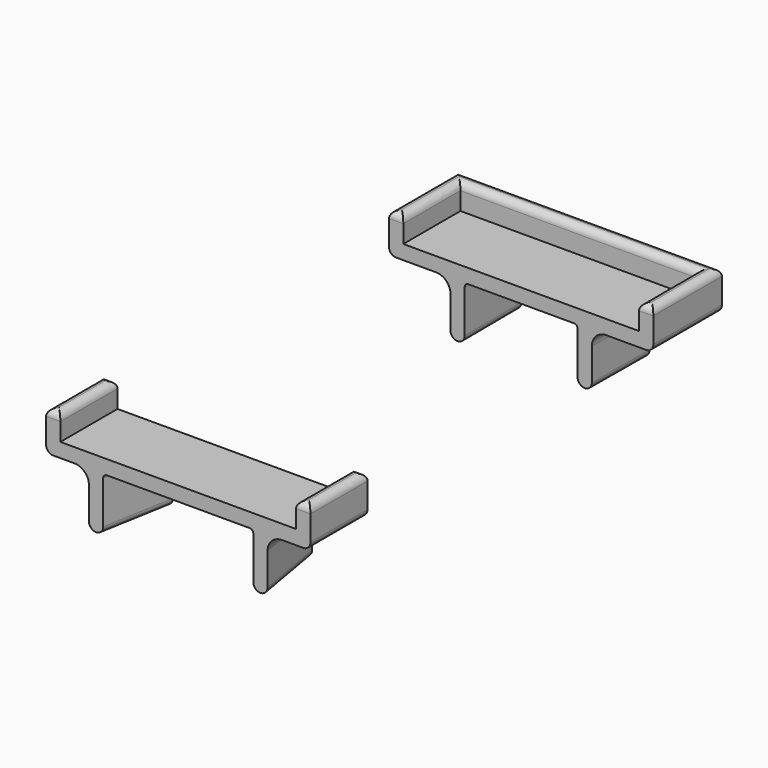
from build123d import *

# Parameters (mm, degrees)
F10_W        = 74
F10_H        = 11
F11_DEPTH    = 4
F12_R        = 1.99999
F12_2_R      = 1.99999
F13_R        = 4
F13_2_R      = 4
F14_R        = 1
F14_2_R      = 1
F15_T1_DEPTH = 30.3039405042
F15_T3_DEPTH = 30.3039405042
F15_T5_DEPTH = 30.3039405042
F15_T7_DEPTH = 30.3039405042
F15_2_F1_R   = 2
F15_2_F2_R   = 1.9999
F15_2_F3_R   = 2
F15_2_F4_R   = 1.9999


# Not quite as in the source:
# - a fillet or chamfer that OpenCascade refuses, or shapes differently, is made with other operations: its cross-section is extruded or revolved along the edge and cut away or added
# - a fillet or chamfer is up to 0.001 mm smaller than in the source, because OpenCascade refuses the exact size


with BuildPart() as f8:
    # F0 (on Front) → F8 section 0
    with BuildSketch(Plane.XZ):
        Polygon((-33, 11), (-37, 11), (-37, 0), (-19.95, 0), (-19.95, -15), (-15.95, -15), (-15.95, 0), (15.95, 0), (15.95, -15), (19.95, -15), (19.95, 0), (37, 0), (37, 11), (33, 11), (33, 4), (-33, 4), align=None)
    # F3 (on plane+point) → F8 section 1
    with BuildSketch(Plane.XZ.offset(20)):
        Polygon((-33, 11), (-37, 11), (-37, 0), (-19.8, 0), (-19.8, -15), (-15.8, -15), (-15.8, 0), (15.8, 0), (15.8, -15), (19.8, -15), (19.8, 0), (37, 0), (37, 11), (33, 11), (33, 4), (-33, 4), align=None)
    loft()

    # F10 (on face) → F11 (join)
    with BuildSketch(Plane(origin=(0, 0, 0), x_dir=(-1, 0, 0), z_dir=(0, 1, 0))):
        with Locations((0, 5.5)):
            Rectangle(F10_W, F10_H)
    extrude(amount=F11_DEPTH)

    # F12 (radius 2 in the source; OpenCascade refuses exactly that, so slightly less here)
    f12_edges = [f8.edges().sort_by_distance(p)[0] for p in [
        (-35, -20, 11),
        (-33, -10, 11),
        (0, 0, 11),
        (33, -10, 11),
        (35, -20, 11),
        (37, -8, 11),
        (0, 4, 11),
        (-37, -8, 11),
        (-37, -8, 0),
        (37, -8, 0),
    ]]
    fillet(f12_edges, radius=F12_R)

    # F13#2
    f13_2_edges = [f8.edges().sort_by_distance(p)[0] for p in [
        (-19.875, -10, 0),
        (19.875, -10, 0),
    ]]
    fillet(f13_2_edges, radius=F13_2_R)

    # F14#2
    f14_2_edges = [f8.edges().sort_by_distance(p)[0] for p in [
        (15.875, -10, 0),
        (-15.875, -10, 0),
    ]]
    fillet(f14_2_edges, radius=F14_2_R)

    # F15#2: fillet of radius 2 on 4 edges, made by hand

    # F15_2_f1
    f15_2_f1_edges = [f8.edges().sort_by_distance(p)[0] for p in [
        (-15.875, -10, -15),
    ]]
    fillet(f15_2_f1_edges, radius=F15_2_F1_R)

    # F15_2_f2 (radius 2 in the source; OpenCascade refuses exactly that, so slightly less here)
    f15_2_f2_edges = [f8.edges().sort_by_distance(p)[0] for p in [
        (-19.875, -10, -15),
    ]]
    fillet(f15_2_f2_edges, radius=F15_2_F2_R)

    # F15_2_f3
    f15_2_f3_edges = [f8.edges().sort_by_distance(p)[0] for p in [
        (15.875, -10, -15),
    ]]
    fillet(f15_2_f3_edges, radius=F15_2_F3_R)

    # F15_2_f4 (radius 2 in the source; OpenCascade refuses exactly that, so slightly less here)
    f15_2_f4_edges = [f8.edges().sort_by_distance(p)[0] for p in [
        (19.875, -10, -15),
    ]]
    fillet(f15_2_f4_edges, radius=F15_2_F4_R)


with BuildPart() as f9:
    # F6 (on plane+point) → F9 section 0
    with BuildSketch(Plane.XZ.offset(120)):
        Polygon((-33, 11), (-37, 11), (-37, 0), (-21.5, 0), (-21.5, -15), (-17.5, -15), (-17.5, 0), (17.5, 0), (17.5, -15), (21.5, -15), (21.5, 0), (37, 0), (37, 11), (33, 11), (33, 4), (-33, 4), align=None)
    # F7 (on plane+point) → F9 section 1
    with BuildSketch(Plane.XZ.offset(140)):
        Polygon((-33, 11), (-37, 11), (-37, 0), (-25, 0), (-25, -15), (-21, -15), (-21, 0), (21, 0), (21, -15), (25, -15), (25, 0), (37, 0), (37, 11), (33, 11), (33, 4), (-33, 4), align=None)
    loft()

    # F12#2 (radius 2 in the source; OpenCascade refuses exactly that, so slightly less here)
    f12_2_edges = [f9.edges().sort_by_distance(p)[0] for p in [
        (-35, -120, 11),
        (-37, -130, 11),
        (-35, -140, 11),
        (-33, -130, 11),
        (35, -120, 11),
        (33, -130, 11),
        (35, -140, 11),
        (37, -130, 11),
        (-37, -130, 0),
        (37, -130, 0),
    ]]
    fillet(f12_2_edges, radius=F12_2_R)

    # F13
    f13_edges = [f9.edges().sort_by_distance(p)[0] for p in [
        (-23.25, -130, 0),
        (23.25, -130, 0),
    ]]
    fillet(f13_edges, radius=F13_R)

    # F14
    f14_edges = [f9.edges().sort_by_distance(p)[0] for p in [
        (-19.25, -130, 0),
        (19.25, -130, 0),
    ]]
    fillet(f14_edges, radius=F14_R)

    # F15: fillet of radius 2 on 4 edges, made by hand

    # F15_s2 → F15_t1 (cut)
    with BuildSketch(Plane(origin=(-20.0340959155, -114.4805480887, 0), x_dir=(0, 0, 1), z_dir=(-0.1723803318, -0.9850304672, 0))):
        with BuildLine():
            ThreePointArc((-13, -3.447606635), (-14.4142135624, -2.8618201974), (-15, -1.447606635))
            Line((-15, -1.447606635), (-15, -3.447606635))
            Line((-15, -3.447606635), (-13, -3.447606635))
        make_face()
    extrude(amount=F15_T1_DEPTH, mode=Mode.SUBTRACT)

    # F15_s4 → F15_t3 (cut)
    with BuildSketch(Plane(origin=(-20.1529558306, -115.1597476036, 0), x_dir=(0, 0, 1), z_dir=(-0.1723803318, -0.9850304672, 0))):
        with BuildLine():
            ThreePointArc((-15, -1.5074847664), (-14.4142135624, -0.093271204), (-13, 0.4925152336))
            Line((-13, 0.4925152336), (-15, 0.4925152336))
            Line((-15, 0.4925152336), (-15, -1.5074847664))
        make_face()
    extrude(amount=F15_T3_DEPTH, mode=Mode.SUBTRACT)

    # F15_s6 → F15_t5 (cut)
    with BuildSketch(Plane(origin=(20.0340959155, -114.4805480887, 0), x_dir=(0, 0, 1), z_dir=(0.1723803318, -0.9850304672, 0))):
        with BuildLine():
            ThreePointArc((-13, 3.447606635), (-14.4142135624, 2.8618201974), (-15, 1.447606635))
            Line((-15, 1.447606635), (-15, 3.447606635))
            Line((-15, 3.447606635), (-13, 3.447606635))
        make_face()
    extrude(amount=F15_T5_DEPTH, mode=Mode.SUBTRACT)

    # F15_s8 → F15_t7 (cut)
    with BuildSketch(Plane(origin=(20.1529558306, -115.1597476036, 0), x_dir=(0, 0, 1), z_dir=(0.1723803318, -0.9850304672, 0))):
        with BuildLine():
            ThreePointArc((-15, 1.5074847664), (-14.4142135624, 0.093271204), (-13, -0.4925152336))
            Line((-13, -0.4925152336), (-15, -0.4925152336))
            Line((-15, -0.4925152336), (-15, 1.5074847664))
        make_face()
    extrude(amount=F15_T7_DEPTH, mode=Mode.SUBTRACT)


solid = Compound([f8.part, f9.part])
